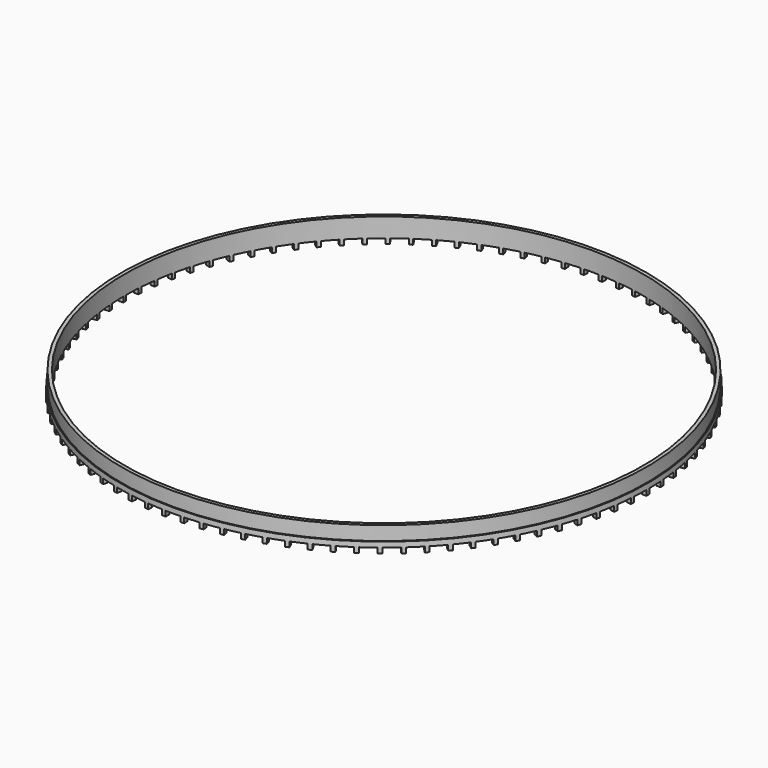
from build123d import *

# Parameters (mm, degrees)
F2_W            = 2.1
F2_H            = 1.5
F3_DEPTH        = 75.651
F3_COPIES_COUNT = 90


# Not quite as in the source:
# - a pattern or mirror of a feature is missing from the dataset's text; its kind, count and spacing are read off the source's solid


with BuildPart() as f1:
    # F0 (on Right) → F1 (revolve)
    with BuildSketch(Plane.YZ):
        Polygon((-75.65, 0), (-74.35, 0), (-74.35, 7), (-75.35, 7), (-75.35, 3), (-75.65, 3), align=None)
    revolve(axis=Axis((0, 0, 3.3058281988), (0, 0, 1)))

    # F2 (on Front) → F3 (cut, through all)
    with BuildSketch(Plane.XZ):
        with Locations((1.05, 0.75)):
            Rectangle(F2_W, F2_H)
        with Locations((-1.05, 0.75)):
            Rectangle(F2_W, F2_H)
    f3 = extrude(amount=-F3_DEPTH, mode=Mode.SUBTRACT)

    # F3_copies: F3 ×90 about axis
    f3_copies_axis = Axis((0, 0, 0), (0, 0, 1))
    for i in range(1, F3_COPIES_COUNT):
        add(f3.rotate(f3_copies_axis, i * 360 / F3_COPIES_COUNT), mode=Mode.SUBTRACT)


solid = f1.part
